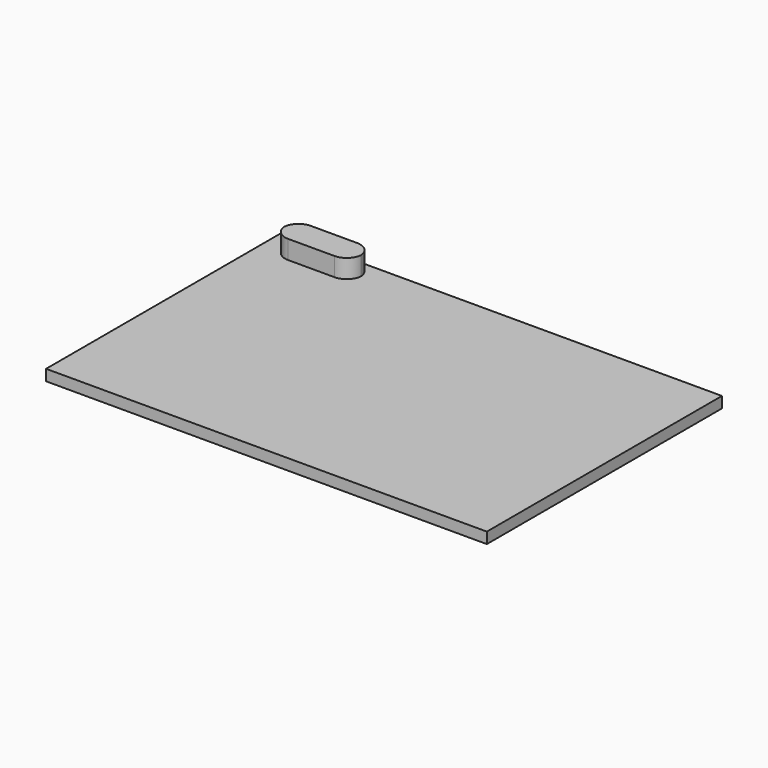
from build123d import *

# Parameters (mm, degrees)
F0_W        = 60
F0_H        = 1.5
F1_DEPTH    = 20
F2_W        = 10.4806274176
F2_H        = 3.8417847827
F3_DEPTH    = 2.54
F4_T1_DEPTH = 7.7522870812


# Not quite as in the source:
# - a fillet or chamfer that OpenCascade refuses, or shapes differently, is made with other operations: its cross-section is extruded or revolved along the edge and cut away or added


with BuildPart() as f1:
    # F0 (on Front) → F1 (new body, symmetric)
    with BuildSketch(Plane.XZ):
        Rectangle(F0_W, F0_H)
    extrude(amount=F1_DEPTH, both=True)

    # F2 (on face) → F3 (join)
    with BuildSketch(Plane.XY.offset(0.75)):
        with Locations((-22.3847124726, 17.5385358743)):
            Rectangle(F2_W, F2_H)
    extrude(amount=F3_DEPTH)

    # F4: fillet of radius 2.0849148325 on 4 edges, made by hand

    # F4_s2 → F4_t1 (cut)
    with BuildSketch(Plane.XY.offset(0.75)):
        with BuildLine():
            ThreePointArc((-27.6250261813, 17.7025583154), (-27.0143687651, 16.2283008992), (-25.5401113489, 15.617643483))
            Line((-25.5401113489, 15.617643483), (-27.6250261813, 15.617643483))
            Line((-27.6250261813, 15.617643483), (-27.6250261813, 17.7025583154))
        make_face()
        with BuildLine():
            ThreePointArc((-25.5401113489, 19.4594282657), (-27.0143687651, 18.8487708495), (-27.6250261813, 17.3745134332))
            Line((-27.6250261813, 17.3745134332), (-27.6250261813, 19.4594282657))
            Line((-27.6250261813, 19.4594282657), (-25.5401113489, 19.4594282657))
        make_face()
        with BuildLine():
            ThreePointArc((-19.2293135962, 15.617643483), (-17.75505618, 16.2283008992), (-17.1443987638, 17.7025583154))
            Line((-17.1443987638, 17.7025583154), (-17.1443987638, 15.617643483))
            Line((-17.1443987638, 15.617643483), (-19.2293135962, 15.617643483))
        make_face()
        with BuildLine():
            ThreePointArc((-19.2293135962, 19.4594282657), (-17.75505618, 18.8487708495), (-17.1443987638, 17.3745134332))
            Line((-17.1443987638, 17.3745134332), (-17.1443987638, 19.4594282657))
            Line((-17.1443987638, 19.4594282657), (-19.2293135962, 19.4594282657))
        make_face()
    extrude(amount=F4_T1_DEPTH, mode=Mode.SUBTRACT)


solid = f1.part
